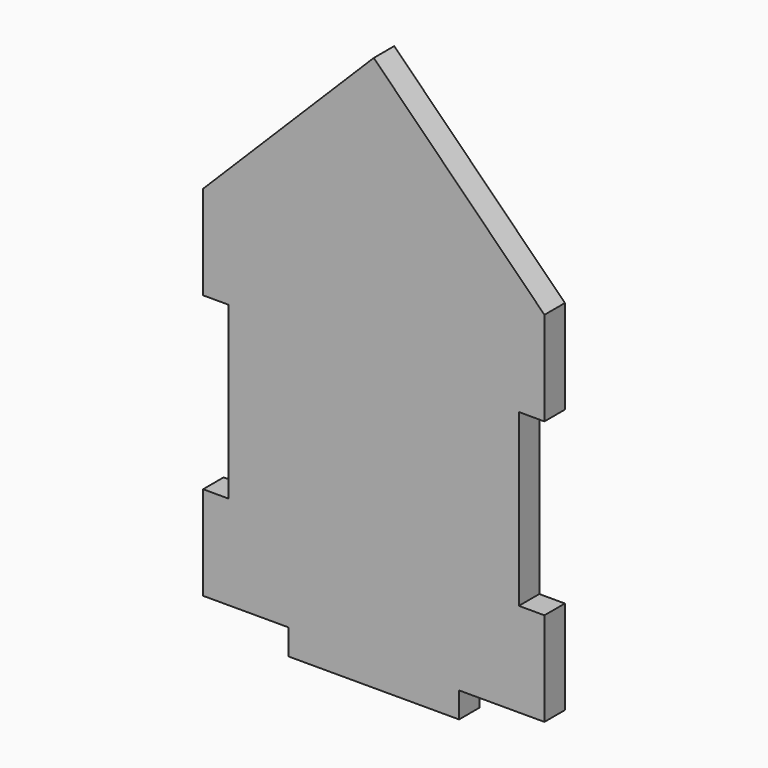
from build123d import *

# Parameters (mm, degrees)
F0_W     = 20
F0_H     = 3
F1_DEPTH = 3


# Not quite as in the source:
# - a feature names something its author has since deleted; it is built from what else it names


with BuildPart() as f1:
    # F0 (on Front) → F1 (new body)
    with BuildSketch(Plane.XZ):
        Polygon((10, -21), (20, -21), (20, -10), (17, -10), (17, 10), (20, 10), (20, 21), (0, 41), (-20, 21), (-20, 10), (-17, 10), (-17, -10), (-20, -10), (-20, -21), (-10, -21), align=None)
        with Locations((0, -22.5)):
            Rectangle(F0_W, F0_H)
    extrude(amount=-F1_DEPTH)


solid = f1.part
